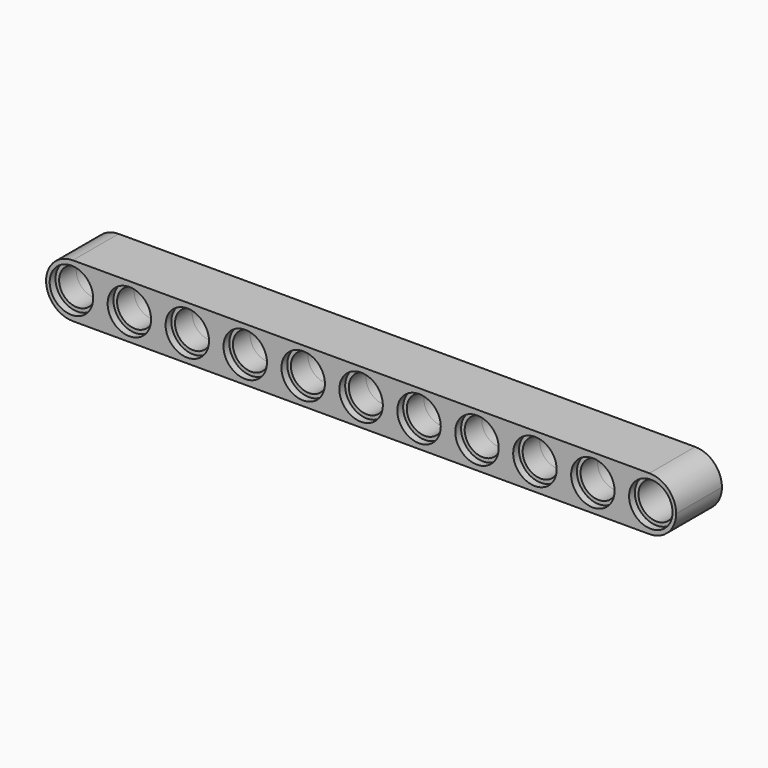
from build123d import *

# Parameters (mm, degrees)
F0_W     = 87
F0_H     = 7.4
F0_R     = 3
F1_DEPTH = 3.95
F0_R_2   = 2.499
F2_DEPTH = 2.95
F3_R     = 3.69999


# Not quite as in the source:
# - a fillet or chamfer is up to 0.001 mm smaller than in the source, because OpenCascade refuses the exact size


with BuildPart() as f1:
    # F0 (on Front) → F1 (new body, symmetric)
    with BuildSketch(Plane.XZ):
        Rectangle(F0_W, F0_H)
        with Locations((-40, 0)):
            Circle(F0_R, mode=Mode.SUBTRACT)
        with Locations((-32, 0)):
            Circle(F0_R, mode=Mode.SUBTRACT)
        with Locations((-24, 0)):
            Circle(F0_R, mode=Mode.SUBTRACT)
        with Locations((-16, 0)):
            Circle(F0_R, mode=Mode.SUBTRACT)
        with Locations((-8, 0)):
            Circle(F0_R, mode=Mode.SUBTRACT)
        Circle(F0_R, mode=Mode.SUBTRACT)
        with Locations((8, 0)):
            Circle(F0_R, mode=Mode.SUBTRACT)
        with Locations((16, 0)):
            Circle(F0_R, mode=Mode.SUBTRACT)
        with Locations((24, 0)):
            Circle(F0_R, mode=Mode.SUBTRACT)
        with Locations((32, 0)):
            Circle(F0_R, mode=Mode.SUBTRACT)
        with Locations((40, 0)):
            Circle(F0_R, mode=Mode.SUBTRACT)
    extrude(amount=F1_DEPTH, both=True)

    # F0 (on Front) → F2 (join, symmetric)
    with BuildSketch(Plane.XZ):
        with Locations((-40, 0)):
            Circle(F0_R)
        with Locations((-40, 0)):
            Circle(F0_R_2, mode=Mode.SUBTRACT)
        with Locations((-32, 0)):
            Circle(F0_R)
        with Locations((-32, 0)):
            Circle(F0_R_2, mode=Mode.SUBTRACT)
        with Locations((-24, 0)):
            Circle(F0_R)
        with Locations((-24, 0)):
            Circle(F0_R_2, mode=Mode.SUBTRACT)
        with Locations((-16, 0)):
            Circle(F0_R)
        with Locations((-16, 0)):
            Circle(F0_R_2, mode=Mode.SUBTRACT)
        with Locations((-8, 0)):
            Circle(F0_R)
        with Locations((-8, 0)):
            Circle(F0_R_2, mode=Mode.SUBTRACT)
        Circle(F0_R)
        Circle(F0_R_2, mode=Mode.SUBTRACT)
        with Locations((8, 0)):
            Circle(F0_R)
        with Locations((8, 0)):
            Circle(F0_R_2, mode=Mode.SUBTRACT)
        with Locations((16, 0)):
            Circle(F0_R)
        with Locations((16, 0)):
            Circle(F0_R_2, mode=Mode.SUBTRACT)
        with Locations((24, 0)):
            Circle(F0_R)
        with Locations((24, 0)):
            Circle(F0_R_2, mode=Mode.SUBTRACT)
        with Locations((32, 0)):
            Circle(F0_R)
        with Locations((32, 0)):
            Circle(F0_R_2, mode=Mode.SUBTRACT)
        with Locations((40, 0)):
            Circle(F0_R)
        with Locations((40, 0)):
            Circle(F0_R_2, mode=Mode.SUBTRACT)
    extrude(amount=F2_DEPTH, both=True)

    # F3 (radius 3.7 in the source; OpenCascade refuses exactly that, so slightly less here)
    f3_edges = [f1.edges().sort_by_distance(p)[0] for p in [
        (-43.5, 0, 3.7),
        (-43.5, 0, -3.7),
        (43.5, 0, 3.7),
        (43.5, 0, -3.7),
    ]]
    fillet(f3_edges, radius=F3_R)


solid = f1.part
